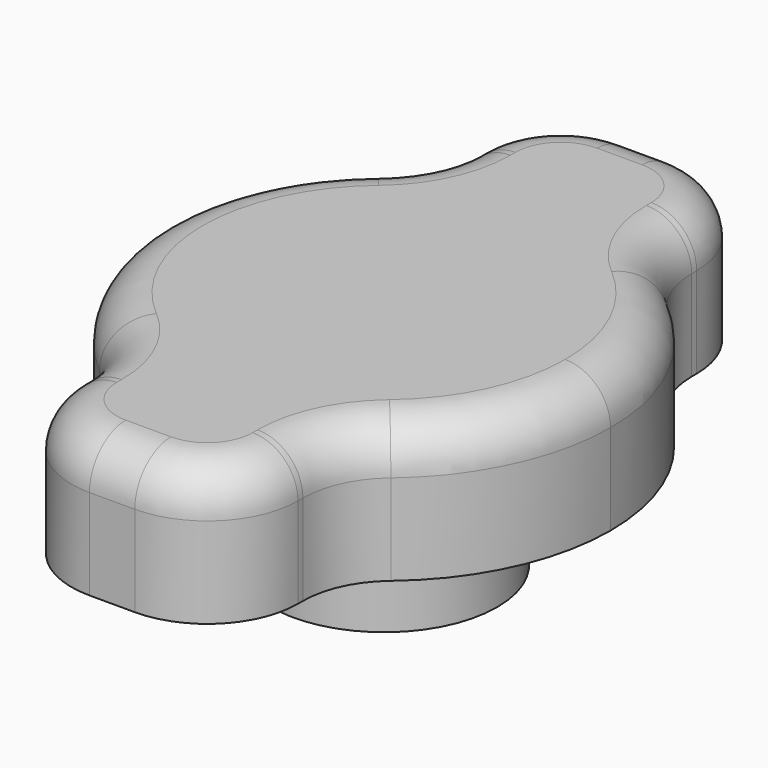
from build123d import *

# Parameters (mm, degrees)
F1_DEPTH = 7.62
F2_R     = 5.08
F3_R     = 2.54
F4_R     = 6.35
F5_DEPTH = 5.842
F7_DEPTH = 11.2014


with BuildPart() as f1:
    # F0 (on Top) → F1 (new body)
    with BuildSketch(Plane.XY):
        with BuildLine():
            ThreePointArc((6.35, -10.9985226281), (10.9985226281, -6.35), (12.7, 0))
            ThreePointArc((12.7, 0), (10.9985226281, 6.35), (6.35, 10.9985226281))
            Line((6.35, 10.9985226281), (6.35, -10.9985226281))
        make_face()
        with BuildLine():
            Line((6.35, -10.9985226281), (6.35, 10.9985226281))
            ThreePointArc((6.35, 10.9985226281), (0, 12.7), (-6.35, 10.9985226281))
            Line((-6.35, 10.9985226281), (-6.35, -10.9985226281))
            ThreePointArc((-6.35, -10.9985226281), (0, -12.7), (6.35, -10.9985226281))
        make_face()
        with BuildLine():
            ThreePointArc((-6.35, 10.9985226281), (0, 12.7), (6.35, 10.9985226281))
            Line((6.35, 10.9985226281), (6.35, 19.05))
            Line((6.35, 19.05), (-6.35, 19.05))
            Line((-6.35, 19.05), (-6.35, 10.9985226281))
        make_face()
        with BuildLine():
            Line((6.35, -19.05), (6.35, -10.9985226281))
            ThreePointArc((6.35, -10.9985226281), (0, -12.7), (-6.35, -10.9985226281))
            Line((-6.35, -10.9985226281), (-6.35, -19.05))
            Line((-6.35, -19.05), (6.35, -19.05))
        make_face()
        with BuildLine():
            Line((-6.35, -10.9985226281), (-6.35, 10.9985226281))
            ThreePointArc((-6.35, 10.9985226281), (-12.7, 0), (-6.35, -10.9985226281))
        make_face()
    extrude(amount=F1_DEPTH)

    # F2
    f2_edges = [f1.edges().sort_by_distance(p)[0] for p in [
        (6.35, -10.998523, 3.81),
        (6.35, -19.05, 3.81),
        (-6.35, -19.05, 3.81),
        (-6.35, -10.998523, 3.81),
        (-6.35, 10.998523, 3.81),
        (-6.35, 19.05, 3.81),
        (6.35, 19.05, 3.81),
        (6.35, 10.998523, 3.81),
    ]]
    fillet(f2_edges, radius=F2_R)

    # F3
    f3_edges = [f1.edges().sort_by_distance(p)[0] for p in [
        (12.7, 0, 7.62),
        (6.825859, -11.472541, 7.62),
        (6.825859, 11.472541, 7.62),
        (6.35, -13.794616, 7.62),
        (6.35, 13.794616, 7.62),
        (4.862102, -17.562102, 7.62),
        (4.862102, 17.562102, 7.62),
        (0, -19.05, 7.62),
        (0, 19.05, 7.62),
        (-4.862102, -17.562102, 7.62),
        (-4.862102, 17.562102, 7.62),
        (-6.35, -13.794616, 7.62),
        (-6.35, 13.794616, 7.62),
        (-6.825859, -11.472541, 7.62),
        (-6.825859, 11.472541, 7.62),
        (-12.7, 0, 7.62),
    ]]
    fillet(f3_edges, radius=F3_R)

    # F4 (on face) → F5 (join)
    with BuildSketch(Plane(origin=(0, 0, 0), x_dir=(1, 0, 0), z_dir=(0, 0, -1))):
        Circle(F4_R)
    extrude(amount=F5_DEPTH)

    # F6 (on face) → F7 (cut)
    with BuildSketch(Plane(origin=(0, 0, -5.842), x_dir=(1, 0, 0), z_dir=(0, 0, -1))):
        with BuildLine():
            Line((-2.1082, 2.3740509177), (-2.1082, -2.3740509177))
            ThreePointArc((-2.1082, -2.3740509177), (3.175, 0), (-2.1082, 2.3740509177))
        make_face()
    extrude(amount=-F7_DEPTH, mode=Mode.SUBTRACT)


solid = f1.part
